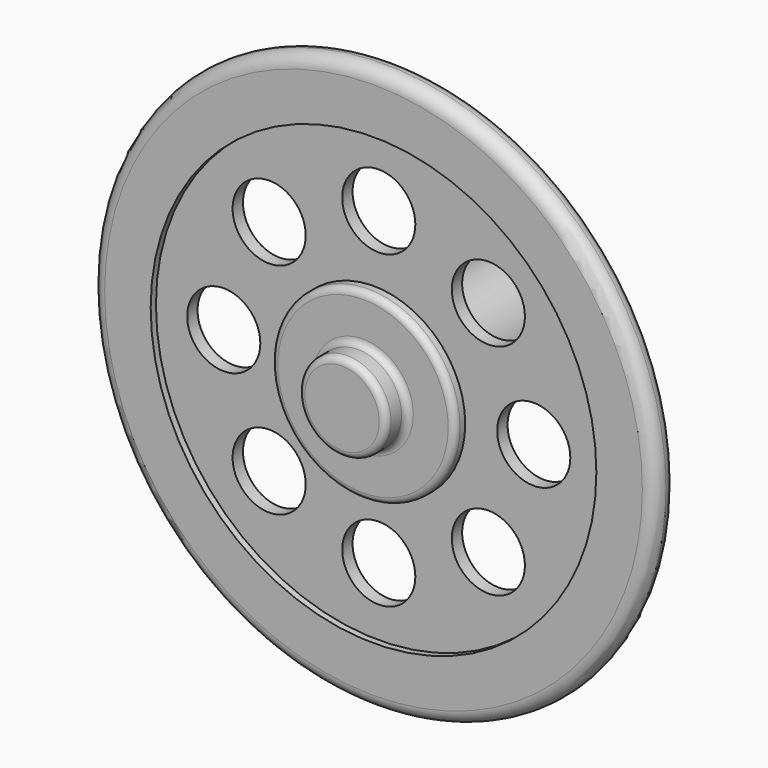
from build123d import *

# Parameters (mm, degrees)
F0_R      = 17.0815
F2_DEPTH  = 1.5875
F3_R      = 5.55625
F4_DEPTH  = 0.79375
F5_R      = 2.6488813199
F6_DEPTH  = 1.5875
F8_R      = 13.5001
F9_DEPTH  = 0.396875
F12_R     = 2.2148075351
F13_DEPTH = 203.2
F14_R     = 3.175
F14_R_2   = 1.5875
F15_DEPTH = 7.9375
F16_R     = 0.79374
F17_R     = 0.396875
F18_R     = 13.5001
F19_DEPTH = 0.4064


# Not quite as in the source:
# - a fillet or chamfer is up to 0.001 mm smaller than in the source, because OpenCascade refuses the exact size
# - a feature of the source that left no trace in its solid (it failed there, or was rolled back) is left out
# - the program builds the solid bodies; features that only make, move or delete a surface that nothing else refers to are left out


with BuildPart() as f2:
    # F0 (on Front) → F2 (new body)
    with BuildSketch(Plane.XZ):
        Circle(F0_R)
    extrude(amount=F2_DEPTH)

    # F3 (on face) → F4 (join)
    with BuildSketch(Plane.XZ.offset(1.5875)):
        Circle(F3_R)
    extrude(amount=F4_DEPTH)

    # F5 (on face) → F6 (join)
    with BuildSketch(Plane.XZ.offset(2.38125)):
        Circle(F5_R)
    extrude(amount=F6_DEPTH)

    # F8 (on face) → F9 (cut)
    with BuildSketch(Plane.XZ.offset(1.5875)):
        Circle(F8_R)
    extrude(amount=-F9_DEPTH, mode=Mode.SUBTRACT)

    # F12 (on face) → F13 (cut)
    with BuildSketch(Plane.XZ.offset(1.5875)):
        with Locations((0, 9.3898363411)):
            Circle(F12_R)
        with Locations((-9.3898363411, 0)):
            Circle(F12_R)
        with Locations((-6.6396169511, 6.6396169511)):
            Circle(F12_R)
        with Locations((-6.6396169511, -6.6396169511)):
            Circle(F12_R)
        with Locations((6.6396169511, 6.6396169511)):
            Circle(F12_R)
        with Locations((9.3898363411, 0)):
            Circle(F12_R)
        with Locations((6.6396169511, -6.6396169511)):
            Circle(F12_R)
        with Locations((0, -9.3898363411)):
            Circle(F12_R)
    extrude(amount=-F13_DEPTH, mode=Mode.SUBTRACT)

    # F14 (on face) → F15 (join)
    with BuildSketch(Plane.XZ):
        Circle(F14_R)
        Circle(F14_R_2, mode=Mode.SUBTRACT)
    extrude(amount=-F15_DEPTH)

    # F16 (radius 0.79375 in the source; OpenCascade refuses exactly that, so slightly less here)
    f16_edges = [f2.edges().sort_by_distance(p)[0] for p in [
        (-17.0815, 0, 0),
        (-17.0815, -1.5875, 0),
        (-3.175, 0, 0),
    ]]
    fillet(f16_edges, radius=F16_R)

    # F17
    f17_edges = [f2.edges().sort_by_distance(p)[0] for p in [
        (-2.648881, -3.96875, 0),
        (-2.648881, -2.38125, 0),
        (-5.55625, -2.38125, 0),
    ]]
    fillet(f17_edges, radius=F17_R)

    # F18 (on face) → F19 (cut)
    with BuildSketch(Plane.XZ):
        Circle(F18_R)
    extrude(amount=F19_DEPTH, mode=Mode.SUBTRACT)


solid = f2.part
